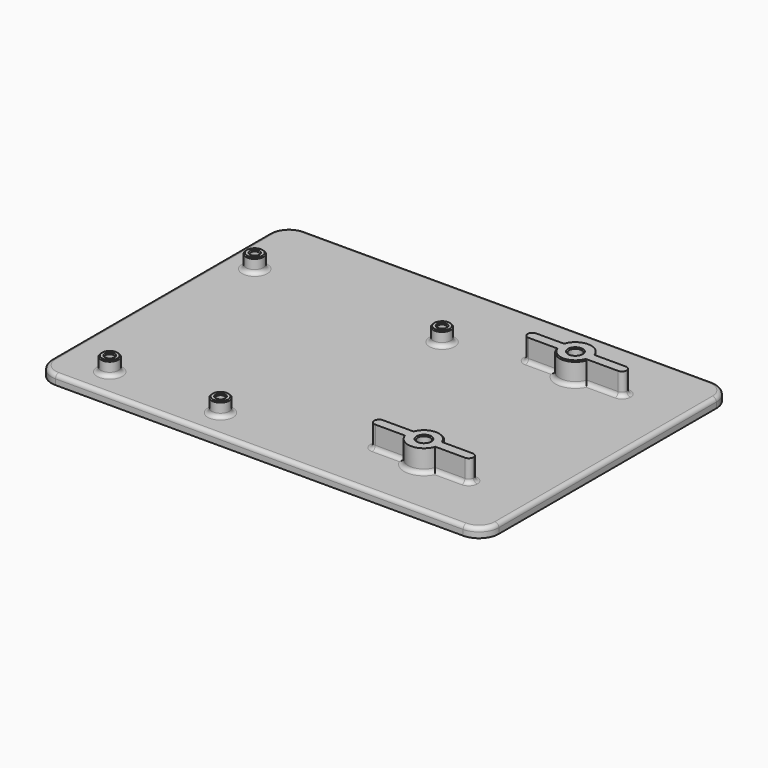
from build123d import *

# Parameters (mm, degrees)
F0_R     = 2.2
F0_R_2   = 1
F1_DEPTH = 6
F0_R_3   = 1.6
F2_DEPTH = 8
F0_W     = 102.79
F0_H     = 68.58
F3_DEPTH = 2.4
F4_SIZE  = 0.25
F5_R     = 1
F6_R     = 1
F7_R     = 1


with BuildPart() as f1:
    # F0 (on Top) → F1 (new body)
    with BuildSketch(Plane.XY):
        with Locations((2.54, 54.61)):
            Circle(F0_R)
        with Locations((2.54, 54.61)):
            Circle(F0_R_2, mode=Mode.SUBTRACT)
    extrude(amount=F1_DEPTH)



with BuildPart() as f1b:
    # F0 (on Top) → F1, piece 2 (new body)
    with BuildSketch(Plane.XY):
        with Locations((7.62, 2.54)):
            Circle(F0_R)
        with Locations((7.62, 2.54)):
            Circle(F0_R_2, mode=Mode.SUBTRACT)
    extrude(amount=F1_DEPTH)


with BuildPart() as f1c:
    # F0 (on Top) → F1, piece 3 (new body)
    with BuildSketch(Plane.XY):
        with Locations((35.56, 2.54)):
            Circle(F0_R)
        with Locations((35.56, 2.54)):
            Circle(F0_R_2, mode=Mode.SUBTRACT)
    extrude(amount=F1_DEPTH)


with BuildPart() as f1d:
    # F0 (on Top) → F1, piece 4 (new body)
    with BuildSketch(Plane.XY):
        with Locations((50.8, 53.34)):
            Circle(F0_R)
        with Locations((50.8, 53.34)):
            Circle(F0_R_2, mode=Mode.SUBTRACT)
    extrude(amount=F1_DEPTH)


with BuildPart() as f2:
    # F0 (on Top) → F2 (new body)
    with BuildSketch(Plane.XY):
        with BuildLine():
            Line((69.7168460011, 56.966), (76.7492431943, 56.966))
            ThreePointArc((76.7492431943, 56.966), (80.565, 54.166), (84.3807568057, 56.966))
            Line((84.3807568057, 56.966), (92.3168460011, 56.966))
            ThreePointArc((92.3168460011, 56.966), (93.1653741386, 57.3174718626), (93.5168460011, 58.166))
            ThreePointArc((93.5168460011, 58.166), (93.1653741386, 59.0145281374), (92.3168460011, 59.366))
            Line((92.3168460011, 59.366), (84.3807568057, 59.366))
            ThreePointArc((84.3807568057, 59.366), (80.565, 62.166), (76.7492431943, 59.366))
            Line((76.7492431943, 59.366), (69.7168460011, 59.366))
            ThreePointArc((69.7168460011, 59.366), (68.8683178637, 59.0145281374), (68.5168460011, 58.166))
            ThreePointArc((68.5168460011, 58.166), (68.8683178637, 57.3174718626), (69.7168460011, 56.966))
        make_face()
        with Locations((80.565, 58.166)):
            Circle(F0_R_3, mode=Mode.SUBTRACT)
    extrude(amount=F2_DEPTH)


with BuildPart() as f2b:
    # F0 (on Top) → F2, piece 2 (new body)
    with BuildSketch(Plane.XY):
        with BuildLine():
            Line((91.865, 11.614), (84.3807568057, 11.614))
            ThreePointArc((84.3807568057, 11.614), (80.565, 14.414), (76.7492431943, 11.614))
            Line((76.7492431943, 11.614), (69.265, 11.614))
            ThreePointArc((69.265, 11.614), (68.4164718626, 11.2625281374), (68.065, 10.414))
            ThreePointArc((68.065, 10.414), (68.4164718626, 9.5654718626), (69.265, 9.214))
            Line((69.265, 9.214), (76.7492431943, 9.214))
            ThreePointArc((76.7492431943, 9.214), (80.565, 6.414), (84.3807568057, 9.214))
            Line((84.3807568057, 9.214), (91.865, 9.214))
            ThreePointArc((91.865, 9.214), (92.7135281374, 9.5654718626), (93.065, 10.414))
            ThreePointArc((93.065, 10.414), (92.7135281374, 11.2625281374), (91.865, 11.614))
        make_face()
        with Locations((80.565, 10.414)):
            Circle(F0_R_3, mode=Mode.SUBTRACT)
    extrude(amount=F2_DEPTH)


with BuildPart() as f1_1:
    add(f1.part)

    add(f1b.part)  # F3 merges F1b

    add(f1c.part)  # F3 merges F1c

    add(f1d.part)  # F3 merges F1d

    add(f2.part)  # F3 merges F2

    add(f2b.part)  # F3 merges F2b
    # F0 (on Top) → F3 (join)
    with BuildSketch(Plane.XY):
        with BuildLine():
            Line((-5, 68.58), (-5, 0))
            ThreePointArc((-5, 0), (-3.5355339059, -3.5355339059), (0, -5))
            Line((0, -5), (102.79, -5))
            ThreePointArc((102.79, -5), (106.3255339059, -3.5355339059), (107.79, 0))
            Line((107.79, 0), (107.79, 68.58))
            ThreePointArc((107.79, 68.58), (106.3255339059, 72.1155339059), (102.79, 73.58))
            Line((102.79, 73.58), (0, 73.58))
            ThreePointArc((0, 73.58), (-3.5355339059, 72.1155339059), (-5, 68.58))
        make_face()
        with Locations((51.395, 34.29)):
            Rectangle(F0_W, F0_H, mode=Mode.SUBTRACT)
        with Locations((51.395, 34.29)):
            Rectangle(F0_W, F0_H)
        with Locations((7.62, 2.54)):
            Circle(F0_R, mode=Mode.SUBTRACT)
        with Locations((35.56, 2.54)):
            Circle(F0_R, mode=Mode.SUBTRACT)
        with BuildLine():
            ThreePointArc((76.7492431943, 11.614), (80.565, 14.414), (84.3807568057, 11.614))
            Line((84.3807568057, 11.614), (91.865, 11.614))
            ThreePointArc((91.865, 11.614), (92.7135281374, 11.2625281374), (93.065, 10.414))
            ThreePointArc((93.065, 10.414), (92.7135281374, 9.5654718626), (91.865, 9.214))
            Line((91.865, 9.214), (84.3807568057, 9.214))
            ThreePointArc((84.3807568057, 9.214), (80.565, 6.414), (76.7492431943, 9.214))
            Line((76.7492431943, 9.214), (69.265, 9.214))
            ThreePointArc((69.265, 9.214), (68.4164718626, 9.5654718626), (68.065, 10.414))
            ThreePointArc((68.065, 10.414), (68.4164718626, 11.2625281374), (69.265, 11.614))
            Line((69.265, 11.614), (76.7492431943, 11.614))
        make_face(mode=Mode.SUBTRACT)
        with Locations((50.8, 53.34)):
            Circle(F0_R, mode=Mode.SUBTRACT)
        with Locations((2.54, 54.61)):
            Circle(F0_R, mode=Mode.SUBTRACT)
        with BuildLine():
            ThreePointArc((84.3807568057, 56.966), (80.565, 54.166), (76.7492431943, 56.966))
            Line((76.7492431943, 56.966), (69.7168460011, 56.966))
            ThreePointArc((69.7168460011, 56.966), (68.8683178637, 57.3174718626), (68.5168460011, 58.166))
            ThreePointArc((68.5168460011, 58.166), (68.8683178637, 59.0145281374), (69.7168460011, 59.366))
            Line((69.7168460011, 59.366), (76.7492431943, 59.366))
            ThreePointArc((76.7492431943, 59.366), (80.565, 62.166), (84.3807568057, 59.366))
            Line((84.3807568057, 59.366), (92.3168460011, 59.366))
            ThreePointArc((92.3168460011, 59.366), (93.1653741386, 59.0145281374), (93.5168460011, 58.166))
            ThreePointArc((93.5168460011, 58.166), (93.1653741386, 57.3174718626), (92.3168460011, 56.966))
            Line((92.3168460011, 56.966), (84.3807568057, 56.966))
        make_face(mode=Mode.SUBTRACT)
    extrude(amount=F3_DEPTH)

    # F4
    f4_edges = [f1_1.edges().sort_by_distance(p)[0] for p in [
        (0.34, 54.61, 6),
        (1.54, 54.61, 6),
        (6.62, 2.54, 6),
        (5.42, 2.54, 6),
        (34.56, 2.54, 6),
        (33.36, 2.54, 6),
        (49.8, 53.34, 6),
        (48.6, 53.34, 6),
        (78.965, 58.166, 8),
        (80.565, 54.166, 8),
        (80.565, 14.414, 8),
        (78.965, 10.414, 8),
    ]]
    chamfer(f4_edges, length=F4_SIZE)

    # F5
    f5_edges = [f1_1.edges().sort_by_distance(p)[0] for p in [
        (0.34, 54.61, 2.4),
    ]]
    fillet(f5_edges, radius=F5_R)

    # F6
    f6_edges = [f1_1.edges().sort_by_distance(p)[0] for p in [
        (5.42, 2.54, 2.4),
        (33.36, 2.54, 2.4),
        (48.6, 53.34, 2.4),
    ]]
    fillet(f6_edges, radius=F6_R)

    # F7
    f7_edges = [f1_1.edges().sort_by_distance(p)[0] for p in [
        (4.42, 2.54, 2.4),
        (-0.66, 54.61, 2.4),
        (-5, 34.29, 2.4),
        (-3.535534, -3.535534, 2.4),
        (51.395, -5, 2.4),
        (106.325534, -3.535534, 2.4),
        (107.79, 34.29, 2.4),
        (106.325534, 72.115534, 2.4),
        (51.395, 73.58, 2.4),
        (-3.535534, 72.115534, 2.4),
        (93.516846, 58.166, 2.4),
        (88.348801, 56.966, 2.4),
        (80.565, 54.166, 2.4),
        (73.233045, 56.966, 2.4),
        (68.516846, 58.166, 2.4),
        (73.233045, 59.366, 2.4),
        (80.565, 62.166, 2.4),
        (88.348801, 59.366, 2.4),
        (73.007122, 11.614, 2.4),
        (80.565, 14.414, 2.4),
        (88.122878, 11.614, 2.4),
        (93.065, 10.414, 2.4),
        (88.122878, 9.214, 2.4),
        (80.565, 6.414, 2.4),
        (73.007122, 9.214, 2.4),
        (68.065, 10.414, 2.4),
        (32.36, 2.54, 2.4),
        (47.6, 53.34, 2.4),
    ]]
    fillet(f7_edges, radius=F7_R)


solid = f1_1.part
